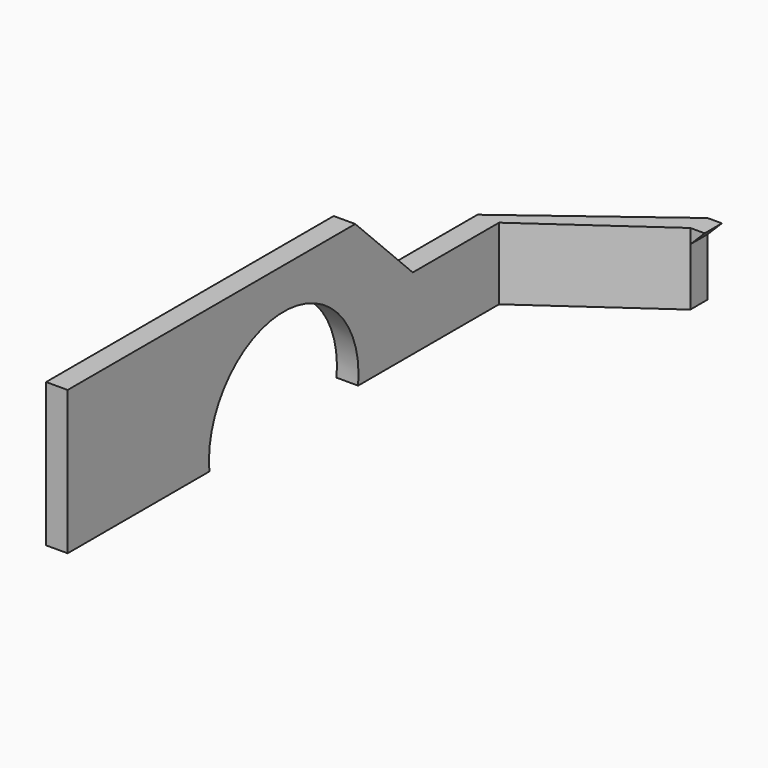
from build123d import *

# Parameters (mm, degrees)
F1_DEPTH = 10
F3_DEPTH = 3
F4_W     = 3
F4_H     = 60
F5_DEPTH = 10
F6_SIZE  = 9.99999
F8_DEPTH = 25


# Not quite as in the source:
# - a fillet or chamfer is up to 0.001 mm smaller than in the source, because OpenCascade refuses the exact size


with BuildPart() as f1:
    # F0 (on Top) → F1 (new body)
    with BuildSketch(Plane.XY):
        Polygon((20, -15), (0, 0), (0, -3), (17, -15), (17, -90), (20, -90), align=None)
    extrude(amount=F1_DEPTH)

    # F2 (on Front) → F3 (join)
    with BuildSketch(Plane.XZ):
        Polygon((0, 8), (0, 10), (-2, 10), align=None)
    extrude(amount=F3_DEPTH)

    # F4 (on face) → F5 (join)
    with BuildSketch(Plane.XY.offset(10)):
        with Locations((18.5, -60)):
            Rectangle(F4_W, F4_H)
    extrude(amount=F5_DEPTH)

    # F6 (size 10 in the source; OpenCascade refuses exactly that, so slightly less here)
    f6_edges = [f1.edges().sort_by_distance(p)[0] for p in [
        (18.5, -30, 20),
    ]]
    chamfer(f6_edges, length=F6_SIZE)

    # F7 (on face) → F8 (cut)
    with BuildSketch(Plane.YZ.offset(20)):
        with BuildLine():
            Line((-65.3636879024, 0), (-39.5, 0))
            ThreePointArc((-39.5, 0), (-52.4318439512, 14.3294404922), (-65.3636879024, 0))
        make_face()
    extrude(amount=-F8_DEPTH, mode=Mode.SUBTRACT)


with BuildPart() as f10_1:
    # F10: instance of F1
    add(f1.part.mirror(Plane.YZ.offset(-2)))


solid = f10_1.part
